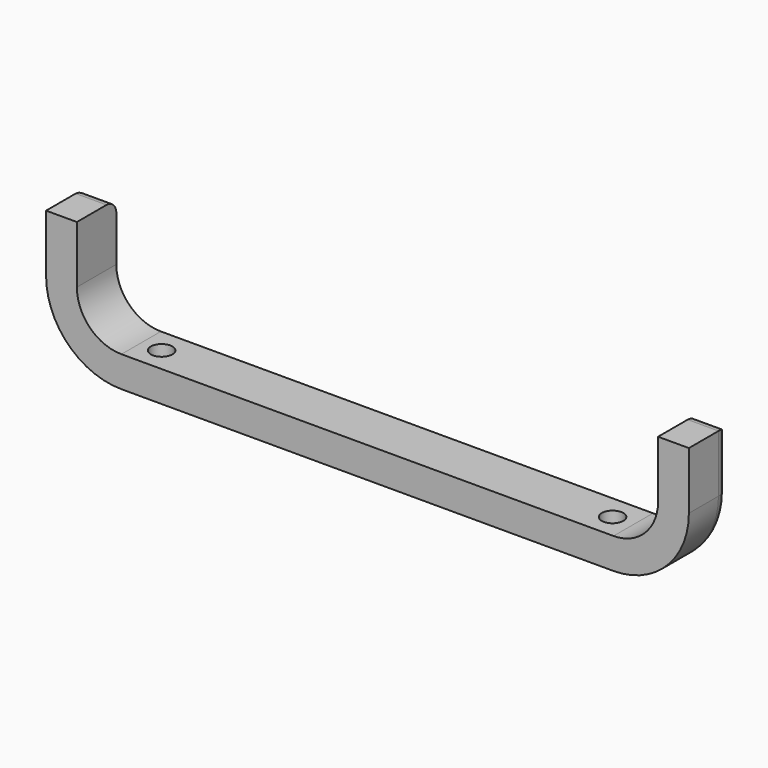
from build123d import *

# Parameters (mm, degrees)
F1_DEPTH       = 5.08
F3_D           = 4.445
F3_CSINK_D     = 7.62
F3_CSINK_ANGLE = 90
F4_T1_DEPTH    = 101.4234647155
F4_T3_DEPTH    = 19.05
F4_T5_DEPTH    = 19.05
F4_T7_DEPTH    = 18.1679810636
F4_T10_ANGLE   = 90
F4_T12_ANGLE   = 90
F5_W           = 25.4
F5_H           = 6.35
F6_DEPTH       = 1.27


# Not quite as in the source:
# - a fillet or chamfer that OpenCascade refuses, or shapes differently, is made with other operations: its cross-section is extruded or revolved along the edge and cut away or added


with BuildPart() as f1:
    # F0 (on Front) → F1 (new body, symmetric)
    with BuildSketch(Plane.XZ):
        with BuildLine():
            Line((50.7117323577, 0), (0, 0))
            Line((0, 0), (-50.7117323577, 0))
            ThreePointArc((-50.7117323577, 0), (-57.2033226337, 2.6889047337), (-59.8922273673, 9.1804950096))
            Line((-59.8922273673, 9.1804950096), (-59.8922273673, 20.9984760731))
            Line((-59.8922273673, 20.9984760731), (-66.2422273673, 20.9984760731))
            Line((-66.2422273673, 20.9984760731), (-66.2422273673, 9.1804950096))
            ThreePointArc((-66.2422273673, 9.1804950096), (-61.6934506942, -1.8012233269), (-50.7117323577, -6.35))
            Line((-50.7117323577, -6.35), (0, -6.35))
            Line((0, -6.35), (50.7117323577, -6.35))
            ThreePointArc((50.7117323577, -6.35), (61.6934506942, -1.8012233269), (66.2422273673, 9.1804950096))
            Line((66.2422273673, 9.1804950096), (66.2422273673, 20.9984760731))
            Line((66.2422273673, 20.9984760731), (59.8922273673, 20.9984760731))
            Line((59.8922273673, 20.9984760731), (59.8922273673, 9.1804950096))
            ThreePointArc((59.8922273673, 9.1804950096), (57.2033226337, 2.6889047337), (50.7117323577, 0))
        make_face()
    extrude(amount=F1_DEPTH, both=True)

    # F3 (through all)
    with Locations(Plane(origin=(0, 0, -6.35), x_dir=(1, 0, 0), z_dir=(0, 0, -1))):
        with Locations((-46.4819967747, 0), (46.443849802, 0)):
            CounterSinkHole(F3_D / 2, F3_CSINK_D / 2, counter_sink_angle=F3_CSINK_ANGLE)

    # F4: fillet of radius 2.54 on 7 edges, made by hand

    # F4_s2 → F4_t1 (cut)
    with BuildSketch(Plane.YZ.offset(-50.7117323577)):
        with BuildLine():
            ThreePointArc((5.08, -3.81), (4.3360512242, -5.6060512242), (2.54, -6.35))
            Line((2.54, -6.35), (5.08, -6.35))
            Line((5.08, -6.35), (5.08, -3.81))
        make_face()
    extrude(amount=F4_T1_DEPTH, mode=Mode.SUBTRACT)

    # F4_s4 → F4_t3 (cut)
    with BuildSketch(Plane.YZ.offset(53.5422273673)):
        with BuildLine():
            ThreePointArc((5.08, 18.4584760731), (4.3360512242, 20.2545272974), (2.54, 20.9984760731))
            Line((2.54, 20.9984760731), (5.08, 20.9984760731))
            Line((5.08, 20.9984760731), (5.08, 18.4584760731))
        make_face()
    extrude(amount=F4_T3_DEPTH, mode=Mode.SUBTRACT)

    # F4_s6 → F4_t5 (cut)
    with BuildSketch(Plane.YZ.offset(-72.5922273673)):
        with BuildLine():
            ThreePointArc((5.08, 18.4584760731), (4.3360512242, 20.2545272974), (2.54, 20.9984760731))
            Line((2.54, 20.9984760731), (5.08, 20.9984760731))
            Line((5.08, 20.9984760731), (5.08, 18.4584760731))
        make_face()
    extrude(amount=F4_T5_DEPTH, mode=Mode.SUBTRACT)

    # F4_s8 → F4_t7 (cut)
    with BuildSketch(Plane.XY.offset(9.1804950096)):
        with BuildLine():
            ThreePointArc((63.7022273673, 5.08), (65.4982785915, 4.3360512242), (66.2422273673, 2.54))
            Line((66.2422273673, 2.54), (66.2422273673, 5.08))
            Line((66.2422273673, 5.08), (63.7022273673, 5.08))
        make_face()
        with BuildLine():
            ThreePointArc((-63.7022273673, 5.08), (-65.4982785915, 4.3360512242), (-66.2422273673, 2.54))
            Line((-66.2422273673, 2.54), (-66.2422273673, 5.08))
            Line((-66.2422273673, 5.08), (-63.7022273673, 5.08))
        make_face()
    extrude(amount=F4_T7_DEPTH, mode=Mode.SUBTRACT)

    # F4_s9 → F4_t10 (revolve, cut)
    with BuildSketch(Plane.YZ.offset(50.7117323577)):
        with BuildLine():
            ThreePointArc((2.54, -6.35), (4.3360512242, -5.6060512242), (5.08, -3.81))
            Line((5.08, -3.81), (5.08, -6.35))
            Line((5.08, -6.35), (2.54, -6.35))
        make_face()
    revolve(axis=Axis((50.7117323577, 5.08, 9.1804950096), (0, -1, 0)), revolution_arc=F4_T10_ANGLE, mode=Mode.SUBTRACT)

    # F4_s11 → F4_t12 (revolve, cut)
    with BuildSketch(Plane.XY.offset(9.1804950096)):
        with BuildLine():
            ThreePointArc((-63.7022273673, 5.08), (-65.4982785915, 4.3360512242), (-66.2422273673, 2.54))
            Line((-66.2422273673, 2.54), (-66.2422273673, 5.08))
            Line((-66.2422273673, 5.08), (-63.7022273673, 5.08))
        make_face()
    revolve(axis=Axis((-50.7117323577, 5.08, 9.1804950096), (0, -1, 0)), revolution_arc=F4_T12_ANGLE, mode=Mode.SUBTRACT)

    # F5 (on face) → F6 (join)
    with BuildSketch(Plane(origin=(0, 0, -6.35), x_dir=(1, 0, 0), z_dir=(0, 0, -1))):
        Rectangle(F5_W, F5_H)
    extrude(amount=F6_DEPTH)


solid = f1.part
